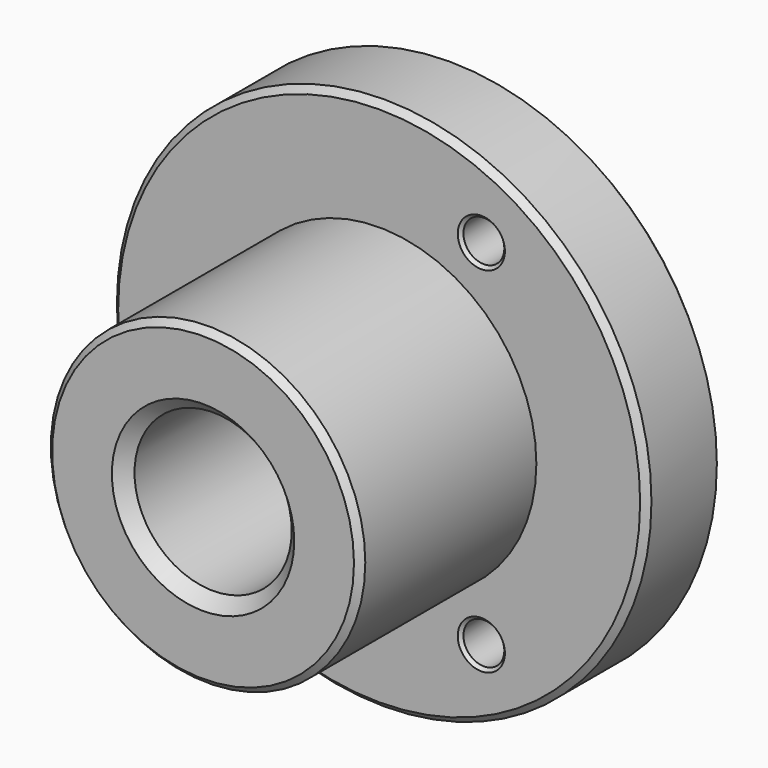
from build123d import *

# Parameters (mm, degrees)
F0_R            = 42.5
F0_R_2          = 25
F1_DEPTH        = 15
F2_DEPTH        = 50
F3_SIZE         = 1
F4_R            = 12.5
F5_DEPTH        = 50.001
F6_SIZE         = 2
F7_R            = 3.25
F8_DEPTH        = 50.001
F8_COPIES_COUNT = 3
F7_R_2          = 6
F9_DEPTH        = 8
F9_COPIES_COUNT = 3
F10_SIZE        = 0.5


# Not quite as in the source:
# - a pattern or mirror of a feature is missing from the dataset's text; its kind, count and spacing are read off the source's solid


with BuildPart() as f1:
    # F0 (on Front) → F1 (new body)
    with BuildSketch(Plane.XZ):
        Circle(F0_R)
        Circle(F0_R_2, mode=Mode.SUBTRACT)
        Circle(F0_R_2)
    extrude(amount=F1_DEPTH)

    # F0 (on Front) → F2 (join)
    with BuildSketch(Plane.XZ):
        Circle(F0_R_2)
    extrude(amount=F2_DEPTH)

    # F3
    f3_edges = [f1.edges().sort_by_distance(p)[0] for p in [
        (-42.5, 0, 0),
        (-42.5, -15, 0),
        (-25, -50, 0),
    ]]
    chamfer(f3_edges, length=F3_SIZE)

    # F4 (on face) → F5 (cut, through all)
    with BuildSketch(Plane.XZ.offset(50)):
        Circle(F4_R)
    extrude(amount=-F5_DEPTH, mode=Mode.SUBTRACT)

    # F6
    f6_edges = [f1.edges().sort_by_distance(p)[0] for p in [
        (-12.5, -50, 0),
        (-12.5, 0, 0),
    ]]
    chamfer(f6_edges, length=F6_SIZE)

    # F7 (on face) → F8 (cut, through all)
    with BuildSketch(Plane(origin=(0, 0, 0), x_dir=(-1, 0, 0), z_dir=(0, 1, 0))):
        with Locations((32.5, 0)):
            Circle(F7_R)
    f8 = extrude(amount=-F8_DEPTH, mode=Mode.SUBTRACT)

    # F8_copies: F8 ×3 about axis
    f8_copies_axis = Axis((0, 0, 0), (0, 1, 0))
    for i in range(1, F8_COPIES_COUNT):
        add(f8.rotate(f8_copies_axis, i * 360 / F8_COPIES_COUNT), mode=Mode.SUBTRACT)

    # F7 (on face) → F9 (cut)
    with BuildSketch(Plane(origin=(0, 0, 0), x_dir=(-1, 0, 0), z_dir=(0, 1, 0))):
        with Locations((32.5, 0)):
            Circle(F7_R_2)
        with Locations((32.5, 0)):
            Circle(F7_R, mode=Mode.SUBTRACT)
    f9 = extrude(amount=-F9_DEPTH, mode=Mode.SUBTRACT)

    # F9_copies: F9 ×3 about axis
    f9_copies_axis = Axis((0, 0, 0), (0, 1, 0))
    for i in range(1, F9_COPIES_COUNT):
        add(f9.rotate(f9_copies_axis, i * 360 / F9_COPIES_COUNT), mode=Mode.SUBTRACT)

    # F10
    f10_edges = [f1.edges().sort_by_distance(p)[0] for p in [
        (-26.5, 0, 0),
        (-29.25, -15, 0),
        (13.25, 0, -22.949673),
        (13.25, 0, 22.949673),
        (14.625, -15, -25.331243),
        (14.625, -15, 25.331243),
    ]]
    chamfer(f10_edges, length=F10_SIZE)


solid = f1.part
